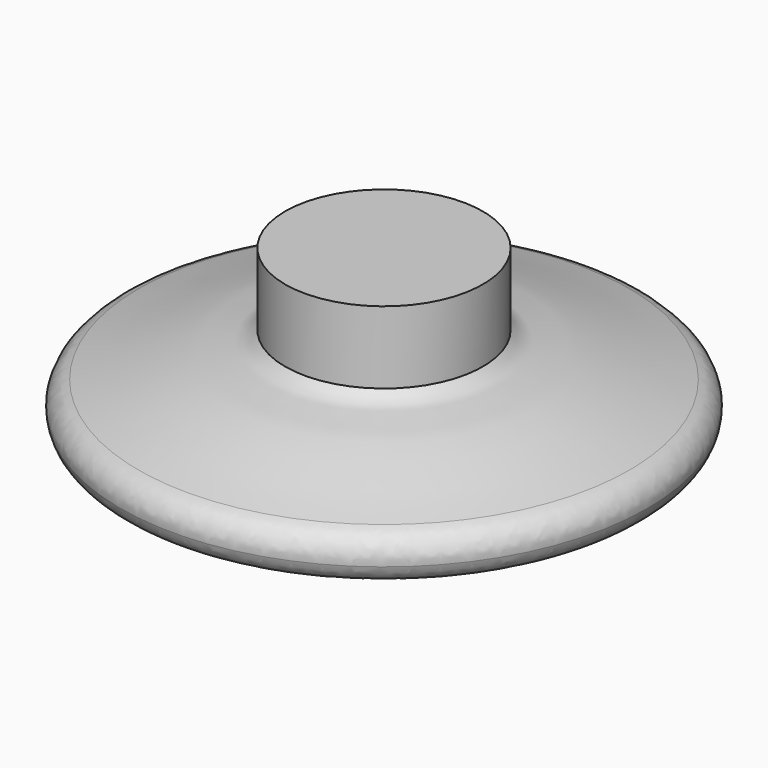
from build123d import *

# Parameters (mm, degrees)
F0_W = 4.1
F0_H = 3
F2_R = 0.99999


# Not quite as in the source:
# - a fillet or chamfer is up to 0.001 mm smaller than in the source, because OpenCascade refuses the exact size
# - the dataset's text gives a spline's control points without its knots; the knots are read off the source's solid


with BuildPart() as f1:
    # F0 (on Front) → F1 (revolve)
    with BuildSketch(Plane.XZ):
        with BuildLine():
            Line((1.0091711268, 2), (-3.0908288732, 2))
            add(Edge.make_bspline(
                [(-3.0908288732, 2), (-3.5489904708, 1.4605779538), (-5.1097833127, 1.6410406807), (-8.02116801, 0.3826504322), (-10.0908288732, 0)],
                knots=[0, 0, 0, 0, 0.3736583672, 1, 1, 1, 1], degree=3))
            Line((-10.0908288732, 0), (-9.7272200714, -1.9666694281))
            add(Edge.make_bspline(
                [(-1.5664662541, 0.7052727679), (-1.742683303, 0.4978015142), (-2.1539394437, 0.1158921106), (-2.8537059622, -0.2527184365), (-3.4709144383, -0.4241706289), (-3.9478517292, -0.4967758357), (-4.2449988158, -0.530522727), (-4.4418275529, -0.5565591275), (-4.5673441131, -0.5761634506), (-4.6998234568, -0.6015656844), (-4.907323153, -0.6475328211), (-5.2083880883, -0.7251991), (-5.6281856313, -0.8471164842), (-6.2540490797, -1.0399729971), (-7.1459267278, -1.3221732356), (-8.3619651623, -1.6736753139), (-9.2590358028, -1.8801089118), (-9.7272200714, -1.9666694281)],
                knots=[0, 0, 0, 0, 0.0625, 0.125, 0.1875, 0.25, 0.3125, 0.34375, 0.375, 0.40625, 0.4375, 0.5, 0.5625, 0.625, 0.75, 0.875, 1, 1, 1, 1], degree=3))
            Line((-1.5664662541, 0.7052727679), (1.0091711268, 2))
        make_face()
        with Locations((-1.0408288732, 3.5)):
            Rectangle(F0_W, F0_H)
    revolve(axis=Axis((1.0091711268, 0, 3.5), (0, 0, 1)))

    # F2 (radius 1 in the source; OpenCascade refuses exactly that, so slightly less here)
    f2_edges = [f1.edges().sort_by_distance(p)[0] for p in [
        (11.745562, 0, -1.966669),
        (12.109171, 0, 0),
    ]]
    fillet(f2_edges, radius=F2_R)


solid = f1.part
